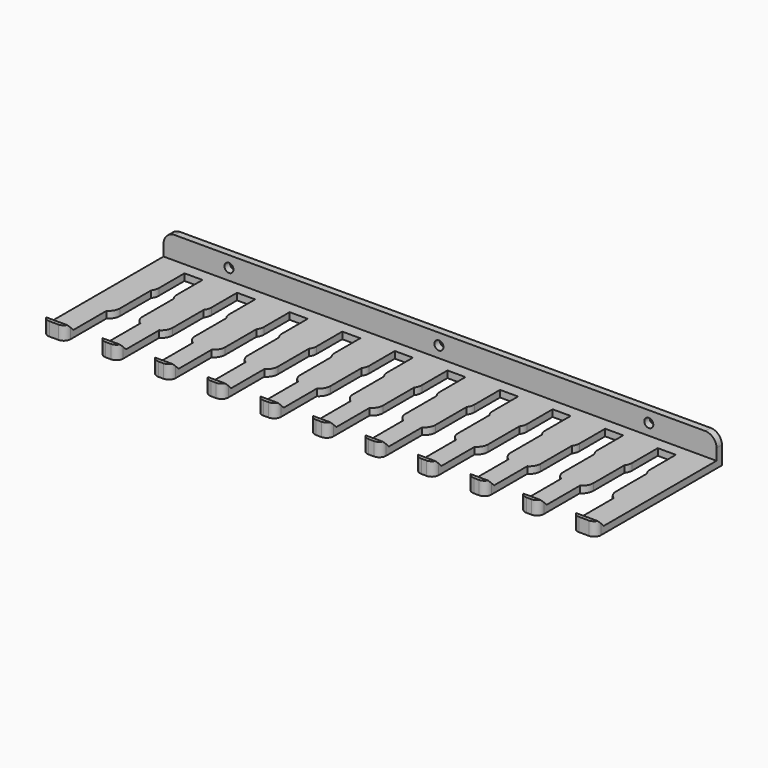
from build123d import *

# Parameters (mm, degrees)
F1_DEPTH     = 3
F2_W         = 245
F2_H         = 2.993311584
F3_DEPTH     = 10
F4_R         = 2
F5_DEPTH     = 25
F6_W         = 10
F6_H         = 8.5889993608
F6_W_2       = 8.3
F6_W_3       = 10.3
F7_DEPTH     = 3
F8_T4_DEPTH  = 44.3035618315
F8_T9_DEPTH  = 46.0035618315
F8_T14_DEPTH = 44.3035618315
F8_T19_DEPTH = 44.3035618315
F8_T24_DEPTH = 44.3035618315
F8_T29_DEPTH = 44.3035618315
F8_T34_DEPTH = 44.3035618315
F8_T39_DEPTH = 44.3035618315
F8_T44_DEPTH = 44.3035618315
F8_T49_DEPTH = 44.3035618315
F8_T54_DEPTH = 46.3035618315
F9_T1_DEPTH  = 18
F9_T3_DEPTH  = 24.6506350946
F10_R        = 3
F11_R        = 5


# Not quite as in the source:
# - a fillet or chamfer that OpenCascade refuses, or shapes differently, is made with other operations: its cross-section is extruded or revolved along the edge and cut away or added


with BuildPart() as f1:
    # F0 (on Top) → F1 (new body)
    with BuildSketch(Plane.XY):
        Polygon((122.5, 35), (-122.5, 35), (-122.5, -35), (-112.5, -35), (-112.5, -12.0593640022), (-110, -12.0593640022), (-110, 9.5146773383), (-109, 9.5146773383), (-109, 26.7303232104), (-101, 26.7303232104), (-101, 9.5146773383), (-100, 9.5146773383), (-100, -12.0593640022), (-97.5, -12.0593640022), (-97.5, -35), (-89.2, -35), (-89.2, -12.0593640022), (-86.7, -12.0593640022), (-86.7, 9.5146773383), (-85.7, 9.5146773383), (-85.7, 26.7303232104), (-77.7, 26.7303232104), (-77.7, 9.5146773383), (-76.7, 9.5146773383), (-76.7, -12.0593640022), (-74.2, -12.0593640022), (-74.2, -35), (-65.9, -35), (-65.9, -12.0593640022), (-63.4, -12.0593640022), (-63.4, 9.5146773383), (-62.4, 9.5146773383), (-62.4, 26.7303232104), (-54.4, 26.7303232104), (-54.4, 9.5146773383), (-53.4, 9.5146773383), (-53.4, -12.0593640022), (-50.9, -12.0593640022), (-50.9, -35), (-42.6, -35), (-42.6, -12.0593640022), (-40.1, -12.0593640022), (-40.1, 9.5146773383), (-39.1, 9.5146773383), (-39.1, 26.7303232104), (-31.1, 26.7303232104), (-31.1, 9.5146773383), (-30.1, 9.5146773383), (-30.1, -12.0593640022), (-27.6, -12.0593640022), (-27.6, -35), (-19.3, -35), (-19.3, -12.0593640022), (-16.8, -12.0593640022), (-16.8, 9.5146773383), (-15.8, 9.5146773383), (-15.8, 26.7303232104), (-7.8, 26.7303232104), (-7.8, 9.5146773383), (-6.8, 9.5146773383), (-6.8, -12.0593640022), (-4.3, -12.0593640022), (-4.3, -35), (4, -35), (4, -12.0593640022), (6.5, -12.0593640022), (6.5, 9.5146773383), (7.5, 9.5146773383), (7.5, 26.7303232104), (15.5, 26.7303232104), (15.5, 9.5146773383), (16.5, 9.5146773383), (16.5, -12.0593640022), (19, -12.0593640022), (19, -35), (27.3, -35), (27.3, -12.0593640022), (29.8, -12.0593640022), (29.8, 9.5146773383), (30.8, 9.5146773383), (30.8, 26.7303232104), (38.8, 26.7303232104), (38.8, 9.5146773383), (39.8, 9.5146773383), (39.8, -12.0593640022), (42.3, -12.0593640022), (42.3, -35), (50.6, -35), (50.6, -12.0593640022), (53.1, -12.0593640022), (53.1, 9.5146773383), (54.1, 9.5146773383), (54.1, 26.7303232104), (62.1, 26.7303232104), (62.1, 9.5146773383), (63.1, 9.5146773383), (63.1, -12.0593640022), (65.6, -12.0593640022), (65.6, -35), (73.9, -35), (73.9, -12.0593640022), (76.4, -12.0593640022), (76.4, 9.5146773383), (77.4, 9.5146773383), (77.4, 26.7303232104), (85.4, 26.7303232104), (85.4, 9.5146773383), (86.4, 9.5146773383), (86.4, -12.0593640022), (88.9, -12.0593640022), (88.9, -35), (97.2, -35), (97.2, -12.0593640022), (99.7, -12.0593640022), (99.7, 9.5146773383), (100.7, 9.5146773383), (100.7, 26.7303232104), (108.7, 26.7303232104), (108.7, 9.5146773383), (109.7, 9.5146773383), (109.7, -12.0593640022), (112.2, -12.0593640022), (112.2, -35), (122.5, -35), align=None)
    extrude(amount=F1_DEPTH)

    # F2 (on face) → F3 (join)
    with BuildSketch(Plane.XY.offset(3)):
        with Locations((0, 33.503344208)):
            Rectangle(F2_W, F2_H)
    extrude(amount=F3_DEPTH)

    # F4 (on face) → F5 (cut)
    with BuildSketch(Plane.XZ.offset(-32.006688416)):
        with Locations((-93.5, 8)):
            Circle(F4_R)
        with Locations((-0.5, 8)):
            Circle(F4_R)
        with Locations((92.5, 8)):
            Circle(F4_R)
    extrude(amount=-F5_DEPTH, mode=Mode.SUBTRACT)

    # F6 (on face) → F7 (join)
    with BuildSketch(Plane.XY.offset(3)):
        with Locations((-117.5, -30.7055003196)):
            Rectangle(F6_W, F6_H)
        with Locations((-93.35, -30.7055003196)):
            Rectangle(F6_W_2, F6_H)
        with Locations((-70.05, -30.7055003196)):
            Rectangle(F6_W_2, F6_H)
        with Locations((-46.75, -30.7055003196)):
            Rectangle(F6_W_2, F6_H)
        with Locations((-23.45, -30.7055003196)):
            Rectangle(F6_W_2, F6_H)
        with Locations((-0.15, -30.7055003196)):
            Rectangle(F6_W_2, F6_H)
        with Locations((23.15, -30.7055003196)):
            Rectangle(F6_W_2, F6_H)
        with Locations((46.45, -30.7055003196)):
            Rectangle(F6_W_2, F6_H)
        with Locations((69.75, -30.7055003196)):
            Rectangle(F6_W_2, F6_H)
        with Locations((93.05, -30.7055003196)):
            Rectangle(F6_W_2, F6_H)
        with Locations((117.35, -30.7055003196)):
            Rectangle(F6_W_3, F6_H)
    extrude(amount=F7_DEPTH)

    # F8: chamfer of 7 on 11 edges, made by hand


with BuildPart() as f8_tool2:
    # F8_s3 → F8_t4 (new body)
    with BuildSketch(Plane.YZ.offset(-71.1982190842)):
        Polygon((-33.4110006392, 6), (-26.4110006392, -1), (-26.4110006392, 6), align=None)
    extrude(amount=-F8_T4_DEPTH)

    split(bisect_by=Plane.XY.offset(3), keep=Keep.TOP)


with BuildPart() as f1_1:
    add(f1.part)

    # F8_t1: cut F8_tool2
    add(f8_tool2.part, mode=Mode.SUBTRACT)


with BuildPart() as f8_tool7:
    # F8_s8 → F8_t9 (new body)
    with BuildSketch(Plane.YZ.offset(-94.4982190842)):
        Polygon((-26.4110006392, -1), (-33.4110006392, 6), (-26.4110006392, 6), align=None)
    extrude(amount=-F8_T9_DEPTH)

    split(bisect_by=Plane.XY.offset(3), keep=Keep.TOP)


with BuildPart() as f1_2:
    add(f1_1.part)

    # F8_t6: cut F8_tool7
    add(f8_tool7.part, mode=Mode.SUBTRACT)


with BuildPart() as f8_tool12:
    # F8_s13 → F8_t14 (new body)
    with BuildSketch(Plane.YZ.offset(-47.8982190842)):
        Polygon((-33.4110006392, 6), (-26.4110006392, -1), (-26.4110006392, 6), align=None)
    extrude(amount=-F8_T14_DEPTH)

    split(bisect_by=Plane.XY.offset(3), keep=Keep.TOP)


with BuildPart() as f1_3:
    add(f1_2.part)

    # F8_t11: cut F8_tool12
    add(f8_tool12.part, mode=Mode.SUBTRACT)


with BuildPart() as f8_tool17:
    # F8_s18 → F8_t19 (new body)
    with BuildSketch(Plane.YZ.offset(-24.5982190842)):
        Polygon((-33.4110006392, 6), (-26.4110006392, -1), (-26.4110006392, 6), align=None)
    extrude(amount=-F8_T19_DEPTH)

    split(bisect_by=Plane.XY.offset(3), keep=Keep.TOP)


with BuildPart() as f1_4:
    add(f1_3.part)

    # F8_t16: cut F8_tool17
    add(f8_tool17.part, mode=Mode.SUBTRACT)


with BuildPart() as f8_tool22:
    # F8_s23 → F8_t24 (new body)
    with BuildSketch(Plane.YZ.offset(-1.2982190842)):
        Polygon((-33.4110006392, 6), (-26.4110006392, -1), (-26.4110006392, 6), align=None)
    extrude(amount=-F8_T24_DEPTH)

    split(bisect_by=Plane.XY.offset(3), keep=Keep.TOP)


with BuildPart() as f1_5:
    add(f1_4.part)

    # F8_t21: cut F8_tool22
    add(f8_tool22.part, mode=Mode.SUBTRACT)


with BuildPart() as f8_tool27:
    # F8_s28 → F8_t29 (new body)
    with BuildSketch(Plane.YZ.offset(22.0017809158)):
        Polygon((-33.4110006392, 6), (-26.4110006392, -1), (-26.4110006392, 6), align=None)
    extrude(amount=-F8_T29_DEPTH)

    split(bisect_by=Plane.XY.offset(3), keep=Keep.TOP)


with BuildPart() as f1_6:
    add(f1_5.part)

    # F8_t26: cut F8_tool27
    add(f8_tool27.part, mode=Mode.SUBTRACT)


with BuildPart() as f8_tool32:
    # F8_s33 → F8_t34 (new body)
    with BuildSketch(Plane.YZ.offset(45.3017809158)):
        Polygon((-33.4110006392, 6), (-26.4110006392, -1), (-26.4110006392, 6), align=None)
    extrude(amount=-F8_T34_DEPTH)

    split(bisect_by=Plane.XY.offset(3), keep=Keep.TOP)


with BuildPart() as f1_7:
    add(f1_6.part)

    # F8_t31: cut F8_tool32
    add(f8_tool32.part, mode=Mode.SUBTRACT)


with BuildPart() as f8_tool37:
    # F8_s38 → F8_t39 (new body)
    with BuildSketch(Plane.YZ.offset(68.6017809158)):
        Polygon((-33.4110006392, 6), (-26.4110006392, -1), (-26.4110006392, 6), align=None)
    extrude(amount=-F8_T39_DEPTH)

    split(bisect_by=Plane.XY.offset(3), keep=Keep.TOP)


with BuildPart() as f1_8:
    add(f1_7.part)

    # F8_t36: cut F8_tool37
    add(f8_tool37.part, mode=Mode.SUBTRACT)


with BuildPart() as f8_tool42:
    # F8_s43 → F8_t44 (new body)
    with BuildSketch(Plane.YZ.offset(91.9017809158)):
        Polygon((-33.4110006392, 6), (-26.4110006392, -1), (-26.4110006392, 6), align=None)
    extrude(amount=-F8_T44_DEPTH)

    split(bisect_by=Plane.XY.offset(3), keep=Keep.TOP)


with BuildPart() as f1_9:
    add(f1_8.part)

    # F8_t41: cut F8_tool42
    add(f8_tool42.part, mode=Mode.SUBTRACT)


with BuildPart() as f8_tool47:
    # F8_s48 → F8_t49 (new body)
    with BuildSketch(Plane.YZ.offset(115.2017809158)):
        Polygon((-33.4110006392, 6), (-26.4110006392, -1), (-26.4110006392, 6), align=None)
    extrude(amount=-F8_T49_DEPTH)

    split(bisect_by=Plane.XY.offset(3), keep=Keep.TOP)


with BuildPart() as f1_10:
    add(f1_9.part)

    # F8_t46: cut F8_tool47
    add(f8_tool47.part, mode=Mode.SUBTRACT)


with BuildPart() as f8_tool52:
    # F8_s53 → F8_t54 (new body)
    with BuildSketch(Plane.YZ.offset(140.5017809158)):
        Polygon((-33.4110006392, 6), (-26.4110006392, -1), (-26.4110006392, 6), align=None)
    extrude(amount=-F8_T54_DEPTH)

    split(bisect_by=Plane.XY.offset(3), keep=Keep.TOP)


with BuildPart() as f1_11:
    add(f1_10.part)

    # F8_t51: cut F8_tool52
    add(f8_tool52.part, mode=Mode.SUBTRACT)

    # F9: fillet of radius 5 on 40 edges, made by hand

    # F9_s2 → F9_t1 (cut)
    with BuildSketch(Plane.XY.offset(-7.5)):
        with BuildLine():
            ThreePointArc((-109, 12.5146773383), (-109.2565835097, 10.9335385082), (-110, 9.5146773383))
            Line((-110, 9.5146773383), (-109, 9.5146773383))
            Line((-109, 9.5146773383), (-109, 12.5146773383))
        make_face()
        with BuildLine():
            ThreePointArc((-85.7, 12.5146773383), (-85.9565835097, 10.9335385082), (-86.7, 9.5146773383))
            Line((-86.7, 9.5146773383), (-85.7, 9.5146773383))
            Line((-85.7, 9.5146773383), (-85.7, 12.5146773383))
        make_face()
        with BuildLine():
            ThreePointArc((-62.4, 12.5146773383), (-62.6565835097, 10.9335385082), (-63.4, 9.5146773383))
            Line((-63.4, 9.5146773383), (-62.4, 9.5146773383))
            Line((-62.4, 9.5146773383), (-62.4, 12.5146773383))
        make_face()
        with BuildLine():
            ThreePointArc((-39.1, 12.5146773383), (-39.3565835097, 10.9335385082), (-40.1, 9.5146773383))
            Line((-40.1, 9.5146773383), (-39.1, 9.5146773383))
            Line((-39.1, 9.5146773383), (-39.1, 12.5146773383))
        make_face()
        with BuildLine():
            ThreePointArc((-15.8, 12.5146773383), (-16.0565835097, 10.9335385082), (-16.8, 9.5146773383))
            Line((-16.8, 9.5146773383), (-15.8, 9.5146773383))
            Line((-15.8, 9.5146773383), (-15.8, 12.5146773383))
        make_face()
        with BuildLine():
            ThreePointArc((7.5, 12.5146773383), (7.2434164903, 10.9335385082), (6.5, 9.5146773383))
            Line((6.5, 9.5146773383), (7.5, 9.5146773383))
            Line((7.5, 9.5146773383), (7.5, 12.5146773383))
        make_face()
        with BuildLine():
            ThreePointArc((30.8, 12.5146773383), (30.5434164903, 10.9335385082), (29.8, 9.5146773383))
            Line((29.8, 9.5146773383), (30.8, 9.5146773383))
            Line((30.8, 9.5146773383), (30.8, 12.5146773383))
        make_face()
        with BuildLine():
            ThreePointArc((54.1, 12.5146773383), (53.8434164903, 10.9335385082), (53.1, 9.5146773383))
            Line((53.1, 9.5146773383), (54.1, 9.5146773383))
            Line((54.1, 9.5146773383), (54.1, 12.5146773383))
        make_face()
        with BuildLine():
            ThreePointArc((77.4, 12.5146773383), (77.1434164903, 10.9335385082), (76.4, 9.5146773383))
            Line((76.4, 9.5146773383), (77.4, 9.5146773383))
            Line((77.4, 9.5146773383), (77.4, 12.5146773383))
        make_face()
        with BuildLine():
            ThreePointArc((100.7, 12.5146773383), (100.4434164903, 10.9335385082), (99.7, 9.5146773383))
            Line((99.7, 9.5146773383), (100.7, 9.5146773383))
            Line((100.7, 9.5146773383), (100.7, 12.5146773383))
        make_face()
        with BuildLine():
            ThreePointArc((-100, 9.5146773383), (-100.7434164903, 10.9335385082), (-101, 12.5146773383))
            Line((-101, 12.5146773383), (-101, 9.5146773383))
            Line((-101, 9.5146773383), (-100, 9.5146773383))
        make_face()
        with BuildLine():
            ThreePointArc((-76.7, 9.5146773383), (-77.4434164903, 10.9335385082), (-77.7, 12.5146773383))
            Line((-77.7, 12.5146773383), (-77.7, 9.5146773383))
            Line((-77.7, 9.5146773383), (-76.7, 9.5146773383))
        make_face()
        with BuildLine():
            ThreePointArc((-53.4, 9.5146773383), (-54.1434164903, 10.9335385082), (-54.4, 12.5146773383))
            Line((-54.4, 12.5146773383), (-54.4, 9.5146773383))
            Line((-54.4, 9.5146773383), (-53.4, 9.5146773383))
        make_face()
        with BuildLine():
            ThreePointArc((-30.1, 9.5146773383), (-30.8434164903, 10.9335385082), (-31.1, 12.5146773383))
            Line((-31.1, 12.5146773383), (-31.1, 9.5146773383))
            Line((-31.1, 9.5146773383), (-30.1, 9.5146773383))
        make_face()
        with BuildLine():
            ThreePointArc((-6.8, 9.5146773383), (-7.5434164903, 10.9335385082), (-7.8, 12.5146773383))
            Line((-7.8, 12.5146773383), (-7.8, 9.5146773383))
            Line((-7.8, 9.5146773383), (-6.8, 9.5146773383))
        make_face()
        with BuildLine():
            ThreePointArc((16.5, 9.5146773383), (15.7565835097, 10.9335385082), (15.5, 12.5146773383))
            Line((15.5, 12.5146773383), (15.5, 9.5146773383))
            Line((15.5, 9.5146773383), (16.5, 9.5146773383))
        make_face()
        with BuildLine():
            ThreePointArc((39.8, 9.5146773383), (39.0565835097, 10.9335385082), (38.8, 12.5146773383))
            Line((38.8, 12.5146773383), (38.8, 9.5146773383))
            Line((38.8, 9.5146773383), (39.8, 9.5146773383))
        make_face()
        with BuildLine():
            ThreePointArc((63.1, 9.5146773383), (62.3565835097, 10.9335385082), (62.1, 12.5146773383))
            Line((62.1, 12.5146773383), (62.1, 9.5146773383))
            Line((62.1, 9.5146773383), (63.1, 9.5146773383))
        make_face()
        with BuildLine():
            ThreePointArc((86.4, 9.5146773383), (85.6565835097, 10.9335385082), (85.4, 12.5146773383))
            Line((85.4, 12.5146773383), (85.4, 9.5146773383))
            Line((85.4, 9.5146773383), (86.4, 9.5146773383))
        make_face()
        with BuildLine():
            ThreePointArc((109.7, 9.5146773383), (108.9565835097, 10.9335385082), (108.7, 12.5146773383))
            Line((108.7, 12.5146773383), (108.7, 9.5146773383))
            Line((108.7, 9.5146773383), (109.7, 9.5146773383))
        make_face()
    extrude(amount=F9_T1_DEPTH, mode=Mode.SUBTRACT)

    # F9_s4 → F9_t3 (cut)
    with BuildSketch(Plane.XY.offset(-10.8253175473)):
        with BuildLine():
            ThreePointArc((-110, -7.7292369833), (-110.6698729811, -10.2292369833), (-112.5, -12.0593640022))
            Line((-112.5, -12.0593640022), (-110, -12.0593640022))
            Line((-110, -12.0593640022), (-110, -7.7292369833))
        make_face()
        with BuildLine():
            ThreePointArc((-86.7, -7.7292369833), (-87.3698729811, -10.2292369833), (-89.2, -12.0593640022))
            Line((-89.2, -12.0593640022), (-86.7, -12.0593640022))
            Line((-86.7, -12.0593640022), (-86.7, -7.7292369833))
        make_face()
        with BuildLine():
            ThreePointArc((-63.4, -7.7292369833), (-64.0698729811, -10.2292369833), (-65.9, -12.0593640022))
            Line((-65.9, -12.0593640022), (-63.4, -12.0593640022))
            Line((-63.4, -12.0593640022), (-63.4, -7.7292369833))
        make_face()
        with BuildLine():
            ThreePointArc((-40.1, -7.7292369833), (-40.7698729811, -10.2292369833), (-42.6, -12.0593640022))
            Line((-42.6, -12.0593640022), (-40.1, -12.0593640022))
            Line((-40.1, -12.0593640022), (-40.1, -7.7292369833))
        make_face()
        with BuildLine():
            ThreePointArc((-16.8, -7.7292369833), (-17.4698729811, -10.2292369833), (-19.3, -12.0593640022))
            Line((-19.3, -12.0593640022), (-16.8, -12.0593640022))
            Line((-16.8, -12.0593640022), (-16.8, -7.7292369833))
        make_face()
        with BuildLine():
            ThreePointArc((6.5, -7.7292369833), (5.8301270189, -10.2292369833), (4, -12.0593640022))
            Line((4, -12.0593640022), (6.5, -12.0593640022))
            Line((6.5, -12.0593640022), (6.5, -7.7292369833))
        make_face()
        with BuildLine():
            ThreePointArc((29.8, -7.7292369833), (29.1301270189, -10.2292369833), (27.3, -12.0593640022))
            Line((27.3, -12.0593640022), (29.8, -12.0593640022))
            Line((29.8, -12.0593640022), (29.8, -7.7292369833))
        make_face()
        with BuildLine():
            ThreePointArc((99.7, -7.7292369833), (99.0301270189, -10.2292369833), (97.2, -12.0593640022))
            Line((97.2, -12.0593640022), (99.7, -12.0593640022))
            Line((99.7, -12.0593640022), (99.7, -7.7292369833))
        make_face()
        with BuildLine():
            ThreePointArc((76.4, -7.7292369833), (75.7301270189, -10.2292369833), (73.9, -12.0593640022))
            Line((73.9, -12.0593640022), (76.4, -12.0593640022))
            Line((76.4, -12.0593640022), (76.4, -7.7292369833))
        make_face()
        with BuildLine():
            ThreePointArc((53.1, -7.7292369833), (52.4301270189, -10.2292369833), (50.6, -12.0593640022))
            Line((50.6, -12.0593640022), (53.1, -12.0593640022))
            Line((53.1, -12.0593640022), (53.1, -7.7292369833))
        make_face()
        with BuildLine():
            ThreePointArc((112.2, -12.0593640022), (110.3698729811, -10.2292369833), (109.7, -7.7292369833))
            Line((109.7, -7.7292369833), (109.7, -12.0593640022))
            Line((109.7, -12.0593640022), (112.2, -12.0593640022))
        make_face()
        with BuildLine():
            ThreePointArc((88.9, -12.0593640022), (87.0698729811, -10.2292369833), (86.4, -7.7292369833))
            Line((86.4, -7.7292369833), (86.4, -12.0593640022))
            Line((86.4, -12.0593640022), (88.9, -12.0593640022))
        make_face()
        with BuildLine():
            ThreePointArc((65.6, -12.0593640022), (63.7698729811, -10.2292369833), (63.1, -7.7292369833))
            Line((63.1, -7.7292369833), (63.1, -12.0593640022))
            Line((63.1, -12.0593640022), (65.6, -12.0593640022))
        make_face()
        with BuildLine():
            ThreePointArc((42.3, -12.0593640022), (40.4698729811, -10.2292369833), (39.8, -7.7292369833))
            Line((39.8, -7.7292369833), (39.8, -12.0593640022))
            Line((39.8, -12.0593640022), (42.3, -12.0593640022))
        make_face()
        with BuildLine():
            ThreePointArc((19, -12.0593640022), (17.1698729811, -10.2292369833), (16.5, -7.7292369833))
            Line((16.5, -7.7292369833), (16.5, -12.0593640022))
            Line((16.5, -12.0593640022), (19, -12.0593640022))
        make_face()
        with BuildLine():
            ThreePointArc((-4.3, -12.0593640022), (-6.1301270189, -10.2292369833), (-6.8, -7.7292369833))
            Line((-6.8, -7.7292369833), (-6.8, -12.0593640022))
            Line((-6.8, -12.0593640022), (-4.3, -12.0593640022))
        make_face()
        with BuildLine():
            ThreePointArc((-27.6, -12.0593640022), (-29.4301270189, -10.2292369833), (-30.1, -7.7292369833))
            Line((-30.1, -7.7292369833), (-30.1, -12.0593640022))
            Line((-30.1, -12.0593640022), (-27.6, -12.0593640022))
        make_face()
        with BuildLine():
            ThreePointArc((-50.9, -12.0593640022), (-52.7301270189, -10.2292369833), (-53.4, -7.7292369833))
            Line((-53.4, -7.7292369833), (-53.4, -12.0593640022))
            Line((-53.4, -12.0593640022), (-50.9, -12.0593640022))
        make_face()
        with BuildLine():
            ThreePointArc((-74.2, -12.0593640022), (-76.0301270189, -10.2292369833), (-76.7, -7.7292369833))
            Line((-76.7, -7.7292369833), (-76.7, -12.0593640022))
            Line((-76.7, -12.0593640022), (-74.2, -12.0593640022))
        make_face()
        with BuildLine():
            ThreePointArc((-97.5, -12.0593640022), (-99.3301270189, -10.2292369833), (-100, -7.7292369833))
            Line((-100, -7.7292369833), (-100, -12.0593640022))
            Line((-100, -12.0593640022), (-97.5, -12.0593640022))
        make_face()
    extrude(amount=F9_T3_DEPTH, mode=Mode.SUBTRACT)

    # F10
    f10_edges = [f1_11.edges().sort_by_distance(p)[0] for p in [
        (-112.5, -35, 3),
        (-122.5, -35, 3),
        (-97.5, -35, 3),
        (-89.2, -35, 3),
        (-74.2, -35, 3),
        (-65.9, -35, 3),
        (-50.9, -35, 3),
        (-42.6, -35, 3),
        (-27.6, -35, 3),
        (-19.3, -35, 3),
        (-4.3, -35, 3),
        (4, -35, 3),
        (19, -35, 3),
        (27.3, -35, 3),
        (42.3, -35, 3),
        (50.6, -35, 3),
        (65.6, -35, 3),
        (73.9, -35, 3),
        (88.9, -35, 3),
        (97.2, -35, 3),
        (112.2, -35, 3),
        (122.5, -35, 3),
    ]]
    fillet(f10_edges, radius=F10_R)

    # F11
    f11_edges = [f1_11.edges().sort_by_distance(p)[0] for p in [
        (-122.5, 33.503344, 13),
        (122.5, 33.503344, 13),
    ]]
    fillet(f11_edges, radius=F11_R)


solid = f1_11.part
